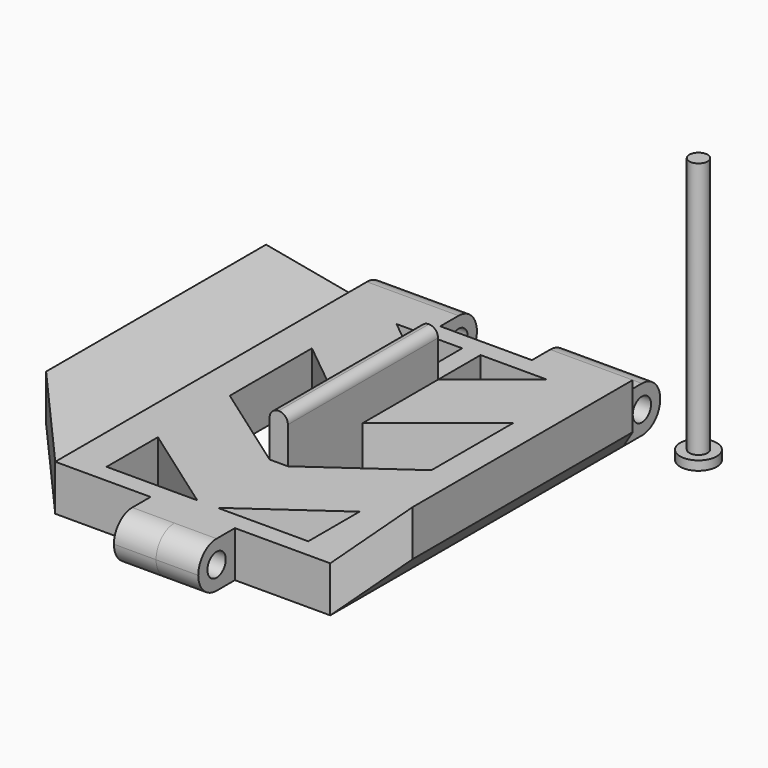
from build123d import *

# Parameters (mm, degrees)
F0_W      = 38.1
F0_H      = 50.8
F1_DEPTH  = 6.35
F3_DEPTH  = 50.8
F4_W      = 25.4
F4_H      = 6.35
F4_R      = 1.5875
F5_DEPTH  = 19.05
F6_W      = 12.7
F6_H      = 3.175
F6_W_2    = 0.508
F7_DEPTH  = 25.4
F9_DEPTH  = 12.7
F13_DEPTH = 6.351
F14_W     = 2.54
F14_H     = 26.006285722
F15_DEPTH = 6.35
F16_R     = 1.26999
F17_R     = 2.54
F18_DEPTH = 1.27
F19_R     = 1.27
F20_DEPTH = 35.56


# Not quite as in the source:
# - a fillet or chamfer is up to 0.001 mm smaller than in the source, because OpenCascade refuses the exact size


with BuildPart() as f1:
    # F0 (on Top) → F1 (new body)
    with BuildSketch(Plane.XY):
        Rectangle(F0_W, F0_H)
    extrude(amount=F1_DEPTH)

    # F2 (on face) → F3 (join, through all)
    with BuildSketch(Plane.XZ.offset(25.4)):
        Polygon((-19.05, 0), (-19.05, 6.35), (-25.4, 12.7), (-25.4, 6.35), align=None)
    extrude(amount=-F3_DEPTH)

    # F4 (on Right) → F5 (join, symmetric)
    with BuildSketch(Plane.YZ):
        with Locations((-12.7, 3.175)):
            Rectangle(F4_W, F4_H)
        with Locations((12.7, 3.175)):
            Rectangle(F4_W, F4_H)
        with BuildLine():
            Line((-28.575, 0), (-25.4, 0))
            Line((-25.4, 0), (-25.4, 6.35))
            Line((-25.4, 6.35), (-28.575, 6.35))
            ThreePointArc((-28.575, 6.35), (-30.8200640303, 5.4200640303), (-31.75, 3.175))
            ThreePointArc((-31.75, 3.175), (-30.8200640303, 0.9299359697), (-28.575, 0))
        make_face()
        with Locations((-28.575, 3.175)):
            Circle(F4_R, mode=Mode.SUBTRACT)
        with BuildLine():
            Line((25.4, 6.35), (25.4, 0))
            Line((25.4, 0), (28.575, 0))
            ThreePointArc((28.575, 0), (30.8200640303, 0.9299359697), (31.75, 3.175))
            ThreePointArc((31.75, 3.175), (30.8200640303, 5.4200640303), (28.575, 6.35))
            Line((28.575, 6.35), (25.4, 6.35))
        make_face()
        with Locations((28.575, 3.175)):
            Circle(F4_R, mode=Mode.SUBTRACT)
    extrude(amount=F5_DEPTH, both=True)

    # F6 (on face) → F7 (cut)
    with BuildSketch(Plane.XY.offset(6.35)):
        with Locations((0, 30.1625)):
            Rectangle(F6_W, F6_H)
        with Locations((0, 26.9875)):
            Rectangle(F6_W, F6_H)
        with Locations((12.7, -30.1625)):
            Rectangle(F6_W, F6_H)
        with Locations((12.7, -26.9875)):
            Rectangle(F6_W, F6_H)
        with Locations((6.096, -26.9875)):
            Rectangle(F6_W_2, F6_H)
        with Locations((6.096, -30.1625)):
            Rectangle(F6_W_2, F6_H)
        with Locations((-12.7, -30.1625)):
            Rectangle(F6_W, F6_H)
        with Locations((-12.7, -26.9875)):
            Rectangle(F6_W, F6_H)
        with Locations((-6.096, -26.9875)):
            Rectangle(F6_W_2, F6_H)
        with Locations((-6.096, -30.1625)):
            Rectangle(F6_W_2, F6_H)
    extrude(amount=-F7_DEPTH, mode=Mode.SUBTRACT)

    # F8 (on face) → F9 (cut, symmetric)
    with BuildSketch(Plane.XY.offset(6.35)):
        Polygon((-35.3634544947, 9.0865455053), (-19.05, 25.4), (-35.675508843, 25.4), align=None)
        Polygon((-34.7037734637, -25.4), (-19.05, -25.4), (-35.0090485041, -9.4409514959), align=None)
    extrude(amount=F9_DEPTH, both=True, mode=Mode.SUBTRACT)

    # F11: F1 across plane


with BuildPart() as f1_1:
    add(f1.part)
    add(f1.part.mirror(Plane(origin=(0, 2.2576834917, 3.175), x_dir=(0, 1, 0), z_dir=(1, 0, 0))))

    # F12 (on face) → F13 (cut, through all)
    with BuildSketch(Plane.XY.offset(6.35)):
        Polygon((-1.27, 22.86), (-10.3751054608, 22.86), (-1.27, 15.4946079875), align=None)
        Polygon((10.3751054608, 22.86), (1.27, 22.86), (1.27, 15.4946079875), align=None)
        Polygon((-1.27, 0), (-13.97, 0), (-13.97, -1.5224442665), (-1.27, -10.5116777345), align=None)
        Polygon((13.97, 0), (1.27, 0), (1.27, -10.5116777345), (13.97, -1.5224442665), align=None)
        Polygon((13.97, -13.97), (1.4101971646, -22.86), (13.97, -22.86), align=None)
        Polygon((-1.4101971646, -22.86), (-13.97, -13.97), (-13.97, -22.86), align=None)
        Polygon((-1.27, 2.4265903223), (-13.97, 12.7), (-13.97, 0), (-1.27, 0), align=None)
        Polygon((1.27, 2.4265903223), (1.27, 0), (13.97, 0), (13.97, 12.7), align=None)
    extrude(amount=-F13_DEPTH, mode=Mode.SUBTRACT)

    # F14 (on face) → F15 (join)
    with BuildSketch(Plane.XY.offset(6.35)):
        with Locations((0, 2.4914651265)):
            Rectangle(F14_W, F14_H)
    extrude(amount=F15_DEPTH)

    # F16 (radius 1.27 in the source; OpenCascade refuses exactly that, so slightly less here)
    f16_edges = [f1_1.edges().sort_by_distance(p)[0] for p in [
        (-1.27, 2.491465, 12.7),
        (1.27, 2.491465, 12.7),
    ]]
    fillet(f16_edges, radius=F16_R)


with BuildPart() as f18:
    # F17 (on face) → F18 (new body)
    with BuildSketch(Plane.XY):
        with Locations((27.4184718728, 27.9149059206)):
            Circle(F17_R)
    extrude(amount=F18_DEPTH)

    # F19 (on face) → F20 (join)
    with BuildSketch(Plane.XY.offset(1.27)):
        with Locations((27.4184718728, 27.9149059206)):
            Circle(F19_R)
    extrude(amount=F20_DEPTH)


solid = Compound([f1_1.part, f18.part])
